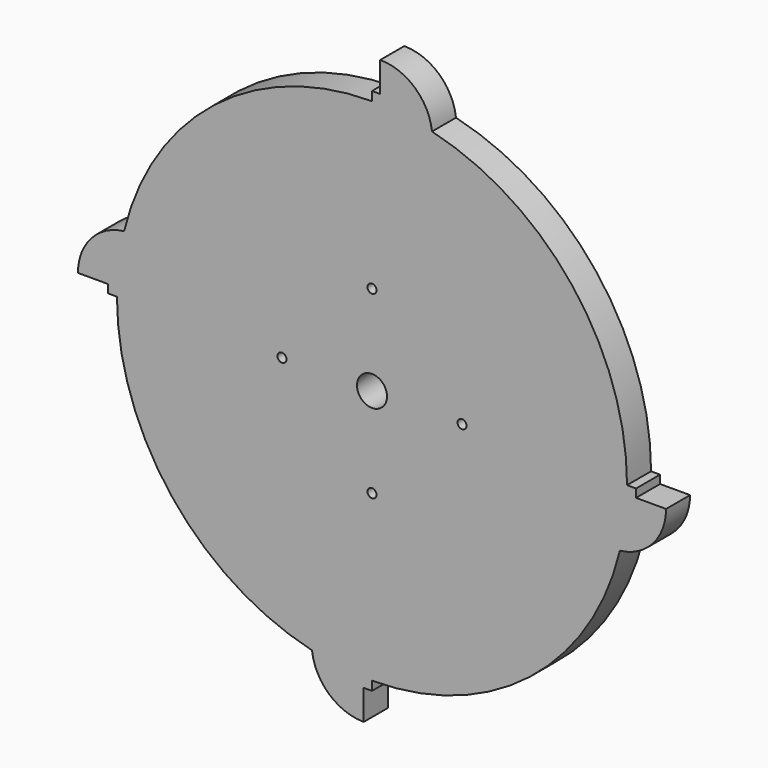
from build123d import *

# Parameters (mm, degrees)
F0_R     = 85
F1_DEPTH = 10
F3_DEPTH = 10
F4_R     = 5
F4_R_2   = 1.5
F5_DEPTH = 10.001


# Not quite as in the source:
# - a feature names something its author has since deleted; it is built from what else it names


with BuildPart() as f1:
    # F0 (on Front) → F1 (new body)
    with BuildSketch(Plane.XZ):
        Circle(F0_R)
    extrude(amount=F1_DEPTH)

    # F2 (on face) → F3 (join)
    with BuildSketch(Plane.XZ.offset(10)):
        with BuildLine():
            Line((0, 88), (0, 85))
            ThreePointArc((0, 85), (10.0709372009, 84.4012809375), (20, 82.6135582093))
            ThreePointArc((20, 82.6135582093), (14.3075201815, 93.5944770544), (2.75, 98))
            Line((2.75, 98), (2.75, 88))
            Line((2.75, 88), (0, 88))
        make_face()
        with BuildLine():
            ThreePointArc((-85, 0), (-84.4012809375, 10.0709372009), (-82.6135582093, 20))
            ThreePointArc((-82.6135582093, 20), (-93.5944770544, 14.3075201815), (-98, 2.75))
            Line((-98, 2.75), (-88, 2.75))
            Line((-88, 2.75), (-88, 0))
            Line((-88, 0), (-85, 0))
        make_face()
        with BuildLine():
            ThreePointArc((0, -85), (-10.0709372009, -84.4012809375), (-20, -82.6135582093))
            ThreePointArc((-20, -82.6135582093), (-14.3075201815, -93.5944770544), (-2.75, -98))
            Line((-2.75, -98), (-2.75, -88))
            Line((-2.75, -88), (0, -88))
            Line((0, -88), (0, -85))
        make_face()
        with BuildLine():
            Line((88, 0), (85, 0))
            ThreePointArc((85, 0), (84.4012809375, -10.0709372009), (82.6135582093, -20))
            ThreePointArc((82.6135582093, -20), (93.5944770544, -14.3075201815), (98, -2.75))
            Line((98, -2.75), (88, -2.75))
            Line((88, -2.75), (88, 0))
        make_face()
    extrude(amount=-F3_DEPTH)

    # F4 (on face) → F5 (cut, through all)
    with BuildSketch(Plane.XZ.offset(10)):
        Circle(F4_R)
        with Locations((0, 30)):
            Circle(F4_R_2)
        with Locations((30, 0)):
            Circle(F4_R_2)
        with Locations((-30, 0)):
            Circle(F4_R_2)
        with Locations((0, -30)):
            Circle(F4_R_2)
    extrude(amount=-F5_DEPTH, mode=Mode.SUBTRACT)


solid = f1.part
